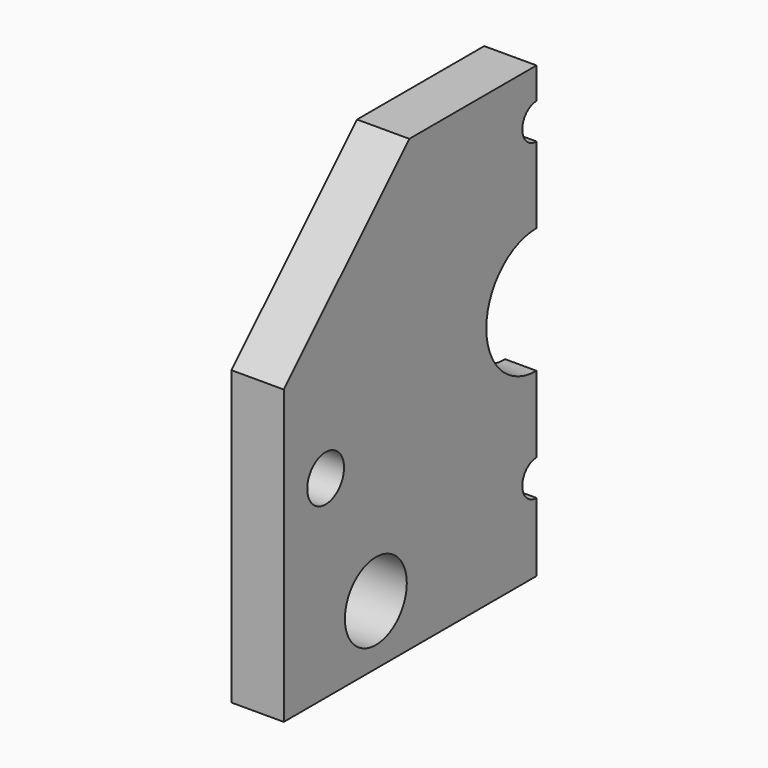
from build123d import *

# Parameters (mm, degrees)
F0_R     = 3.7
F0_R_2   = 2.2
F1_DEPTH = 5
F2_DEPTH = 3
F3_DEPTH = 3
F5_DEPTH = 2


# Not quite as in the source:
# - a feature of the source that left no trace in its solid (it failed there, or was rolled back) is left out


with BuildPart() as f1:
    # F0 (on Right) → F1 (new body)
    with BuildSketch(Plane.YZ):
        with BuildLine():
            Line((-63.5704365752, 33.3448962937), (-63.5704365752, 5.3711892086))
            Line((-63.5704365752, 5.3711892086), (-33.3704365752, 5.3711892086))
            Line((-33.3704365752, 5.3711892086), (-33.3704365752, 11.9448962937))
            ThreePointArc((-33.3704365752, 11.9448962937), (-35.0704365752, 13.6448962937), (-33.3704365752, 15.3448962937))
            Line((-33.3704365752, 15.3448962937), (-33.3704365752, 20.1448962937))
            ThreePointArc((-33.3704365752, 20.1448962937), (-41.8704365752, 28.6448962937), (-33.3704365752, 37.1448962937))
            Line((-33.3704365752, 37.1448962937), (-33.3704365752, 41.9448962937))
            ThreePointArc((-33.3704365752, 41.9448962937), (-35.0704365752, 43.6448962937), (-33.3704365752, 45.3448962937))
            Line((-33.3704365752, 45.3448962937), (-33.3704365752, 48.3448962937))
            Line((-33.3704365752, 48.3448962937), (-48.5704365752, 48.3448962937))
            Line((-48.5704365752, 48.3448962937), (-63.5704365752, 33.3448962937))
        make_face()
        with Locations((-52.5704365752, 11.0711892086)):
            Circle(F0_R, mode=Mode.SUBTRACT)
        with Locations((-58.5704365752, 23.8448962937)):
            Circle(F0_R_2, mode=Mode.SUBTRACT)
        with BuildLine():
            ThreePointArc((-33.3704365752, 37.1448962937), (-41.8704365752, 28.6448962937), (-33.3704365752, 20.1448962937))
            Line((-33.3704365752, 20.1448962937), (-33.3704365752, 22.6448962937))
            ThreePointArc((-33.3704365752, 22.6448962937), (-39.3704365752, 28.6448962937), (-33.3704365752, 34.6448962937))
            Line((-33.3704365752, 34.6448962937), (-33.3704365752, 37.1448962937))
        make_face()
    extrude(amount=F1_DEPTH)

    # F0 (on Right) → F2 (join)
    with BuildSketch(Plane.YZ):
        with BuildLine():
            Line((-63.5704365752, 33.3448962937), (-63.5704365752, 5.3711892086))
            Line((-63.5704365752, 5.3711892086), (-33.3704365752, 5.3711892086))
            Line((-33.3704365752, 5.3711892086), (-33.3704365752, 11.9448962937))
            ThreePointArc((-33.3704365752, 11.9448962937), (-35.0704365752, 13.6448962937), (-33.3704365752, 15.3448962937))
            Line((-33.3704365752, 15.3448962937), (-33.3704365752, 20.1448962937))
            ThreePointArc((-33.3704365752, 20.1448962937), (-41.8704365752, 28.6448962937), (-33.3704365752, 37.1448962937))
            Line((-33.3704365752, 37.1448962937), (-33.3704365752, 41.9448962937))
            ThreePointArc((-33.3704365752, 41.9448962937), (-35.0704365752, 43.6448962937), (-33.3704365752, 45.3448962937))
            Line((-33.3704365752, 45.3448962937), (-33.3704365752, 48.3448962937))
            Line((-33.3704365752, 48.3448962937), (-48.5704365752, 48.3448962937))
            Line((-48.5704365752, 48.3448962937), (-63.5704365752, 33.3448962937))
        make_face()
        with Locations((-52.5704365752, 11.0711892086)):
            Circle(F0_R, mode=Mode.SUBTRACT)
        with Locations((-58.5704365752, 23.8448962937)):
            Circle(F0_R_2, mode=Mode.SUBTRACT)
        with BuildLine():
            ThreePointArc((-33.3704365752, 15.3448962937), (-35.0704365752, 13.6448962937), (-33.3704365752, 11.9448962937))
            Line((-33.3704365752, 11.9448962937), (-33.3704365752, 15.3448962937))
        make_face()
        with BuildLine():
            ThreePointArc((-33.3704365752, 37.1448962937), (-41.8704365752, 28.6448962937), (-33.3704365752, 20.1448962937))
            Line((-33.3704365752, 20.1448962937), (-33.3704365752, 22.6448962937))
            ThreePointArc((-33.3704365752, 22.6448962937), (-39.3704365752, 28.6448962937), (-33.3704365752, 34.6448962937))
            Line((-33.3704365752, 34.6448962937), (-33.3704365752, 37.1448962937))
        make_face()
        with BuildLine():
            Line((-33.3704365752, 41.9448962937), (-33.3704365752, 45.3448962937))
            ThreePointArc((-33.3704365752, 45.3448962937), (-35.0704365752, 43.6448962937), (-33.3704365752, 41.9448962937))
        make_face()
        with BuildLine():
            ThreePointArc((-33.3704365752, 34.6448962937), (-39.3704365752, 28.6448962937), (-33.3704365752, 22.6448962937))
            Line((-33.3704365752, 22.6448962937), (-33.3704365752, 34.6448962937))
        make_face()
    extrude(amount=F2_DEPTH)

    # F0 (on Right) → F3 (cut, through all)
    with BuildSketch(Plane.YZ):
        with BuildLine():
            ThreePointArc((-33.3704365752, 34.6448962937), (-39.3704365752, 28.6448962937), (-33.3704365752, 22.6448962937))
            Line((-33.3704365752, 22.6448962937), (-33.3704365752, 34.6448962937))
        make_face()
        with BuildLine():
            Line((-33.3704365752, 41.9448962937), (-33.3704365752, 45.3448962937))
            ThreePointArc((-33.3704365752, 45.3448962937), (-35.0704365752, 43.6448962937), (-33.3704365752, 41.9448962937))
        make_face()
        with BuildLine():
            ThreePointArc((-33.3704365752, 15.3448962937), (-35.0704365752, 13.6448962937), (-33.3704365752, 11.9448962937))
            Line((-33.3704365752, 11.9448962937), (-33.3704365752, 15.3448962937))
        make_face()
    extrude(amount=F3_DEPTH, mode=Mode.SUBTRACT)

    # F0 (on Right) → F5 (cut)
    with BuildSketch(Plane.YZ):
        with BuildLine():
            ThreePointArc((-33.3704365752, 37.1448962937), (-41.8704365752, 28.6448962937), (-33.3704365752, 20.1448962937))
            Line((-33.3704365752, 20.1448962937), (-33.3704365752, 22.6448962937))
            ThreePointArc((-33.3704365752, 22.6448962937), (-39.3704365752, 28.6448962937), (-33.3704365752, 34.6448962937))
            Line((-33.3704365752, 34.6448962937), (-33.3704365752, 37.1448962937))
        make_face()
    extrude(amount=F5_DEPTH, mode=Mode.SUBTRACT)


solid = f1.part
